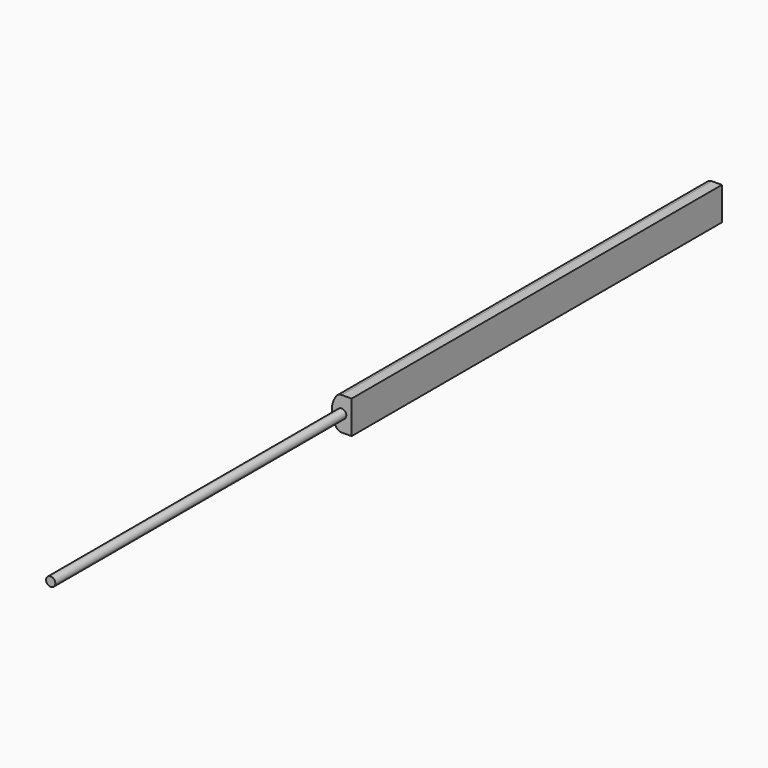
from build123d import *

# Parameters (mm, degrees)
F0_R     = 0.7
F1_DEPTH = 55
F3_DEPTH = 70


# Not quite as in the source:
# - a feature of the source that left no trace in its solid (it failed there, or was rolled back) is left out


with BuildPart() as f1:
    # F0 (on Front) → F1 (new body)
    with BuildSketch(Plane.XZ):
        Circle(F0_R)
    extrude(amount=F1_DEPTH)

    # F2 (on Front) → F3 (join)
    with BuildSketch(Plane.XZ):
        with BuildLine():
            Line((1.5, -2.5), (1.5, 2.5))
            Line((1.5, 2.5), (0, 2.5))
            ThreePointArc((0, 2.5), (-0.4472135955, 2.394427191), (-0.8, 2.1))
            ThreePointArc((-0.8, 2.1), (-1.5, 0), (-0.8, -2.1))
            ThreePointArc((-0.8, -2.1), (-0.4472135955, -2.394427191), (0, -2.5))
            Line((0, -2.5), (1.5, -2.5))
        make_face()
    extrude(amount=-F3_DEPTH)


solid = f1.part
